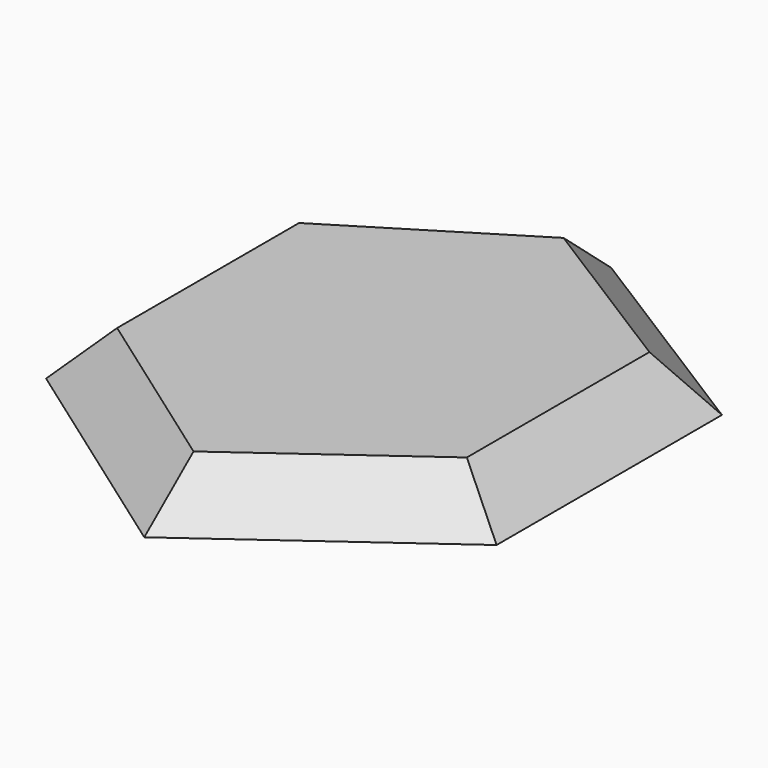
from build123d import *

# Parameters (mm, degrees)
F1_DEPTH    = 0.508
F2_DEPTH    = 3.048
F3_T1_DEPTH = 47.7471989741
F3_T3_DEPTH = 47.4709696523
F3_T5_DEPTH = 47.6607350592
F3_T7_DEPTH = 46.5501838511
F3_T9_DEPTH = 46.8386979916


# Not quite as in the source:
# - a fillet or chamfer that OpenCascade refuses, or shapes differently, is made with other operations: its cross-section is extruded or revolved along the edge and cut away or added


with BuildPart() as f1:
    # F0 (on Top) → F1 (new body)
    with BuildSketch(Plane.XY):
        Polygon((-17.6225993782, 12.5228120014), (0, 0), (17.2826144844, 12.5228120014), (17.2826144844, 34.0552479029), (0, 44.934798032), (-17.6225993782, 34.0552479029), align=None)
    extrude(amount=F1_DEPTH)

    # F2 (add): a face of the model
    f2_faces = [f1.faces().sort_by_distance(p)[0] for p in [
        (-0.1500416402, 22.8299999891, 0.508),
    ]]
    extrude(f2_faces, amount=F2_DEPTH)

    # F3: chamfer of 5.08 on 6 edges, made by hand

    # F3_s2 → F3_t1 (cut)
    with BuildSketch(Plane(origin=(-28.2718126223, 20.0902594906, 0), x_dir=(0, 0, 1), z_dir=(0.8151478349, -0.5792529735, 0))):
        Polygon((-1.524, 0), (3.556, -5.08), (3.556, 0), align=None)
    extrude(amount=F3_T1_DEPTH, mode=Mode.SUBTRACT)

    # F3_s4 → F3_t3 (cut)
    with BuildSketch(Plane(origin=(-10.5789320411, -7.6653898197, 0), x_dir=(0, 0, 1), z_dir=(0.8097681351, 0.5867500042, 0))):
        Polygon((-1.524, 0), (3.556, -5.08), (3.556, 0), align=None)
    extrude(amount=F3_T3_DEPTH, mode=Mode.SUBTRACT)

    # F3_s6 → F3_t5 (cut)
    with BuildSketch(Plane.XZ.offset(-47.1193974817)):
        Polygon((17.2826144844, -1.524), (12.2026144844, 3.556), (17.2826144844, 3.556), align=None)
        Polygon((-12.5425993782, 3.556), (-17.6225993782, -1.524), (-17.6225993782, 3.556), align=None)
    extrude(amount=F3_T5_DEPTH, mode=Mode.SUBTRACT)

    # F3_s8 → F3_t7 (cut)
    with BuildSketch(Plane(origin=(8.0798332195, -5.0863224789, 0), x_dir=(0, 0, 1), z_dir=(-0.846279114, 0.5327397688, 0))):
        Polygon((-1.524, 38.0273810661), (3.556, 32.9473810661), (3.556, 38.0273810661), align=None)
    extrude(amount=F3_T7_DEPTH, mode=Mode.SUBTRACT)

    # F3_s10 → F3_t9 (cut)
    with BuildSketch(Plane(origin=(31.2020521098, 19.2630089793, 0), x_dir=(0, 0, 1), z_dir=(-0.850905843, -0.5253182334, 0))):
        Polygon((-1.524, 38.2352821986), (3.556, 33.1552821986), (3.556, 38.2352821986), align=None)
    extrude(amount=F3_T9_DEPTH, mode=Mode.SUBTRACT)


solid = f1.part
